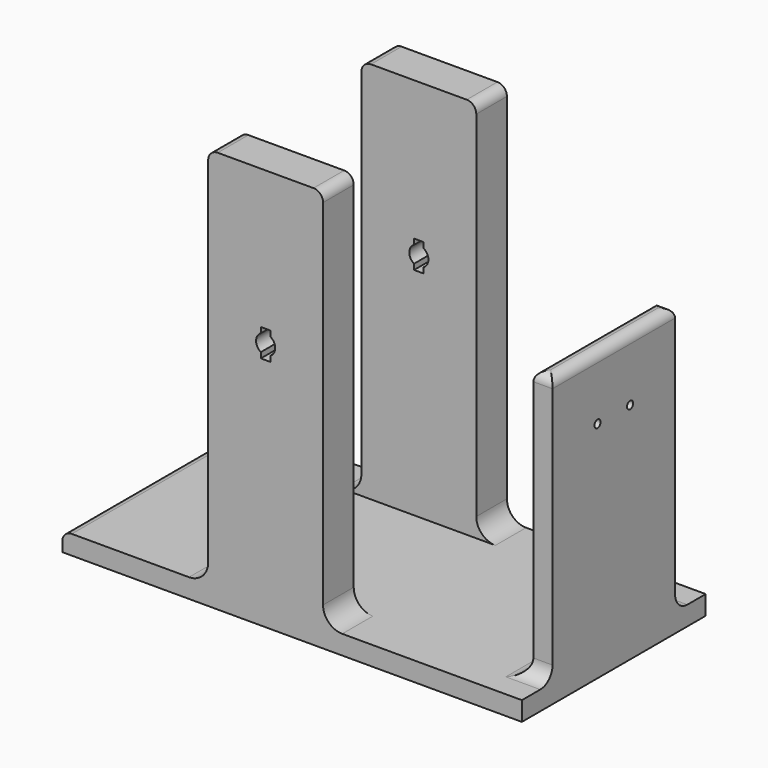
from build123d import *

# Parameters (mm, degrees)
F1_DEPTH = 76.2
F4_DEPTH = 50.8
F7_D     = 2.54
F6_W     = 12.7
F6_H     = 88.9
F8_DEPTH = 6.35
F9_R     = 5.08
F10_R    = 3.17499


# Not quite as in the source:
# - a fillet or chamfer is up to 0.001 mm smaller than in the source, because OpenCascade refuses the exact size


with BuildPart() as f1:
    # F0 (on Front) → F1 (new body)
    with BuildSketch(Plane.XZ):
        with BuildLine():
            Line((-74.9020473927, -80.410034281), (-74.9020473927, -83.585034281))
            Line((-74.9020473927, -83.585034281), (77.4979526073, -83.585034281))
            Line((77.4979526073, -83.585034281), (77.4979526073, -77.235034281))
            Line((77.4979526073, -77.235034281), (77.4979526073, 11.664965719))
            Line((77.4979526073, 11.664965719), (71.1479526073, 11.664965719))
            Line((71.1479526073, 11.664965719), (71.1479526073, -77.235034281))
            Line((71.1479526073, -77.235034281), (17.9289044716, -77.235034281))
            ThreePointArc((17.9289044716, -77.235034281), (13.4387764111, -75.3751623415), (11.5789044716, -70.885034281))
            Line((11.5789044716, -70.885034281), (11.5789044716, 46.589965719))
            ThreePointArc((11.5789044716, 46.589965719), (10.6489685019, 48.8350297493), (8.4039044716, 49.764965719))
            Line((8.4039044716, 49.764965719), (-23.3460955284, 49.764965719))
            ThreePointArc((-23.3460955284, 49.764965719), (-25.5911595586, 48.8350297493), (-26.5210955284, 46.589965719))
            Line((-26.5210955284, 46.589965719), (-26.5210955284, -70.885034281))
            ThreePointArc((-26.5210955284, -70.885034281), (-28.3809674678, -75.3751623415), (-32.8710955284, -77.235034281))
            Line((-32.8710955284, -77.235034281), (-71.7270473927, -77.235034281))
            ThreePointArc((-71.7270473927, -77.235034281), (-73.972111423, -78.1649702507), (-74.9020473927, -80.410034281))
        make_face()
        with BuildLine():
            ThreePointArc((-9.0585955284, -3.784664938), (-10.6460955284, -1.035034281), (-9.0585955284, 1.714596376))
            Line((-9.0585955284, 1.714596376), (-9.0585955284, 3.553124576))
            Line((-9.0585955284, 3.553124576), (-5.8835955284, 3.553124576))
            Line((-5.8835955284, 3.553124576), (-5.8835955284, 1.714596376))
            ThreePointArc((-5.8835955284, 1.714596376), (-4.2960955284, -1.035034281), (-5.8835955284, -3.784664938))
            Line((-5.8835955284, -3.784664938), (-5.8835955284, -5.623193138))
            Line((-5.8835955284, -5.623193138), (-9.0585955284, -5.623193138))
            Line((-9.0585955284, -5.623193138), (-9.0585955284, -3.784664938))
        make_face(mode=Mode.SUBTRACT)
    extrude(amount=F1_DEPTH)

    # F3 (on offset) → F4 (cut, through all)
    with BuildSketch(Plane(origin=(0, -12.7, 0), x_dir=(-1, 0, 0), z_dir=(0, 1, 0))):
        with BuildLine():
            Line((-17.9289044716, -77.235034281), (32.8710955284, -77.235034281))
            ThreePointArc((32.8710955284, -77.235034281), (28.3809674678, -75.3751623415), (26.5210955284, -70.885034281))
            Line((26.5210955284, -70.885034281), (26.5210955284, 46.589965719))
            ThreePointArc((26.5210955284, 46.589965719), (25.5911595586, 48.8350297493), (23.3460955284, 49.764965719))
            Line((23.3460955284, 49.764965719), (-8.4039044716, 49.764965719))
            ThreePointArc((-8.4039044716, 49.764965719), (-10.6489685019, 48.8350297493), (-11.5789044716, 46.589965719))
            Line((-11.5789044716, 46.589965719), (-11.5789044716, -70.885034281))
            ThreePointArc((-11.5789044716, -70.885034281), (-13.4387764111, -75.3751623415), (-17.9289044716, -77.235034281))
        make_face()
    extrude(amount=-F4_DEPTH, mode=Mode.SUBTRACT)

    # F7 (through all)
    with Locations(Plane.YZ.offset(77.4979526073)):
        with Locations((-44.846875, -9.3153121099), (-31.353125, -9.3153121099)):
            Hole(F7_D / 2)

    # F6 (on offset) → F8 (cut)
    with BuildSketch(Plane.YZ.offset(77.4979526073)):
        with Locations((-69.85, -32.785034281)):
            Rectangle(F6_W, F6_H)
        with Locations((-6.35, -32.785034281)):
            Rectangle(F6_W, F6_H)
    extrude(amount=-F8_DEPTH, mode=Mode.SUBTRACT)

    # F9
    f9_edges = [f1.edges().sort_by_distance(p)[0] for p in [
        (74.322953, -12.7, -77.235034),
        (71.147953, -38.1, -77.235034),
        (74.322953, -63.5, -77.235034),
    ]]
    fillet(f9_edges, radius=F9_R)

    # F10 (radius 3.175 in the source; OpenCascade refuses exactly that, so slightly less here)
    f10_edges = [f1.edges().sort_by_distance(p)[0] for p in [
        (74.322953, -63.5, 11.664966),
        (74.322953, -12.7, 11.664966),
        (77.497953, -38.1, 11.664966),
        (71.147953, -38.1, 11.664966),
    ]]
    fillet(f10_edges, radius=F10_R)


solid = f1.part
